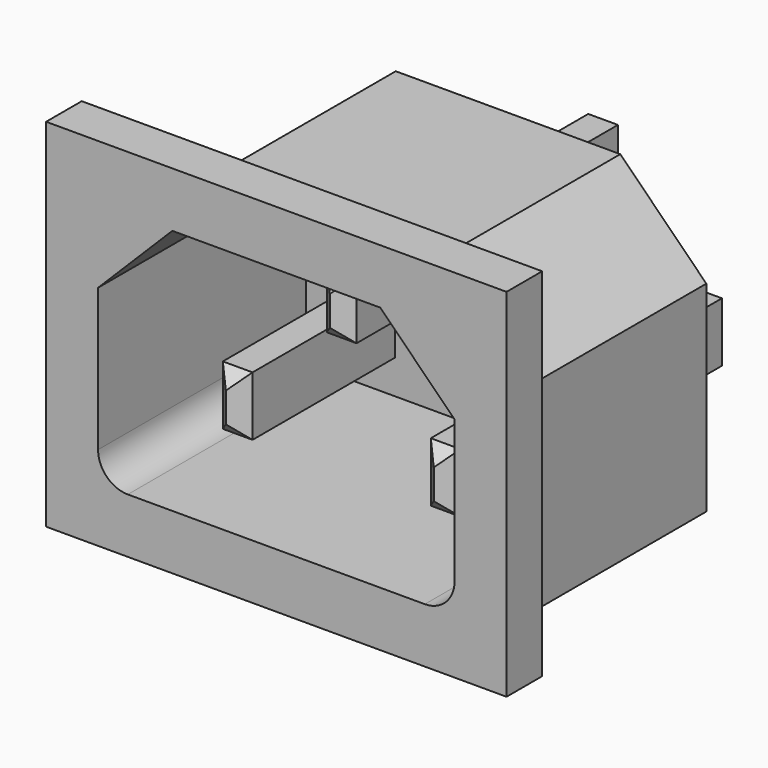
from build123d import *

# Parameters (mm, degrees)
F0_W          = 31
F0_H          = 24
F1_DEPTH      = 3
F3_DEPTH      = 16.5
F5_DEPTH      = 2
F6_W          = 2
F6_H          = 4
F7_DEPTH      = 8
F7_DEPTH_BACK = 15
F8_SIZE       = 0.99999


# Not quite as in the source:
# - a fillet or chamfer is up to 0.001 mm smaller than in the source, because OpenCascade refuses the exact size


with BuildPart() as f1:
    # F0 (on Front) → F1 (new body)
    with BuildSketch(Plane.XZ):
        Rectangle(F0_W, F0_H)
        with BuildLine():
            Line((10, -8.3), (-10, -8.3))
            ThreePointArc((-10, -8.3), (-11.4142135624, -7.7142135624), (-12, -6.3))
            Line((-12, -6.3), (-12, 3.3))
            Line((-12, 3.3), (-7, 8.3))
            Line((-7, 8.3), (7, 8.3))
            Line((7, 8.3), (12, 3.3))
            Line((12, 3.3), (12, -6.3))
            ThreePointArc((12, -6.3), (11.4142135624, -7.7142135624), (10, -8.3))
        make_face(mode=Mode.SUBTRACT)
    extrude(amount=F1_DEPTH)

    # F2 (on face) → F3 (join)
    with BuildSketch(Plane(origin=(0, 0, 0), x_dir=(-1, 0, 0), z_dir=(0, 1, 0))):
        Polygon((-7.5591883092, 9.65), (-13.35, 3.8591883092), (-13.35, -9.65), (13.35, -9.65), (13.35, 3.8591883092), (7.5591883092, 9.65), align=None)
        with BuildLine():
            Line((-12, -6.3), (-12, 3.3))
            Line((-12, 3.3), (-7, 8.3))
            Line((-7, 8.3), (7, 8.3))
            Line((7, 8.3), (12, 3.3))
            Line((12, 3.3), (12, -6.3))
            ThreePointArc((12, -6.3), (11.4142135624, -7.7142135624), (10, -8.3))
            Line((10, -8.3), (-10, -8.3))
            ThreePointArc((-10, -8.3), (-11.4142135624, -7.7142135624), (-12, -6.3))
        make_face(mode=Mode.SUBTRACT)
    extrude(amount=F3_DEPTH)

    # F4 (on face) → F5 (join)
    with BuildSketch(Plane(origin=(0, 16.5, 0), x_dir=(-1, 0, 0), z_dir=(0, 1, 0))):
        Polygon((7.5591883092, 9.65), (-7.5591883092, 9.65), (-13.35, 3.8591883092), (-13.35, -9.65), (13.35, -9.65), (13.35, 3.8591883092), align=None)
    extrude(amount=-F5_DEPTH)

    # F6 (on face) → F7 (join, two sides)
    with BuildSketch(Plane(origin=(0, 16.5, 0), x_dir=(-1, 0, 0), z_dir=(0, 1, 0))) as f7_sk:
        with Locations((0, 4)):
            Rectangle(F6_W, F6_H)
        with Locations((7, -4)):
            Rectangle(F6_W, F6_H)
        with Locations((-7, -4)):
            Rectangle(F6_W, F6_H)
    extrude(amount=F7_DEPTH)
    extrude(f7_sk.sketch, amount=-F7_DEPTH_BACK)

    # F8 (size 1 in the source; OpenCascade refuses exactly that, so slightly less here)
    f8_edges = [f1.edges().sort_by_distance(p)[0] for p in [
        (0, 1.5, 2),
        (-1, 1.5, 4),
        (0, 1.5, 6),
        (1, 1.5, 4),
        (8, 1.5, -4),
        (7, 1.5, -6),
        (6, 1.5, -4),
        (7, 1.5, -2),
        (-7, 1.5, -6),
        (-8, 1.5, -4),
        (-7, 1.5, -2),
        (-6, 1.5, -4),
    ]]
    chamfer(f8_edges, length=F8_SIZE)


solid = f1.part
